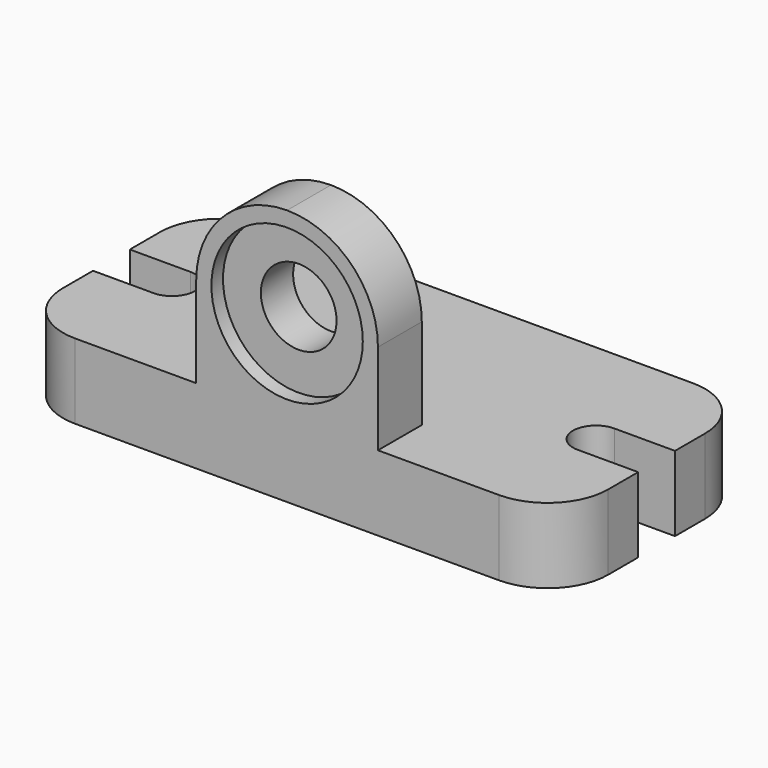
from build123d import *

# Parameters (mm, degrees)
F1_DEPTH = 15.748
F2_W     = 38.1
F2_H     = 11.4949838928
F3_DEPTH = 38.1
F4_R     = 19.04999
F6_D     = 15.875
F7_R     = 15.875
F7_R_2   = 7.9375
F8_DEPTH = 3.048


# Not quite as in the source:
# - a fillet or chamfer is up to 0.001 mm smaller than in the source, because OpenCascade refuses the exact size


with BuildPart() as f1:
    # F0 (on Top) → F1 (new body)
    with BuildSketch(Plane.XY):
        with BuildLine():
            Line((-30.7737162879, 0), (58.1262837121, 0))
            ThreePointArc((58.1262837121, 0), (67.1065398331, 3.7197438789), (70.8262837121, 12.7))
            Line((70.8262837121, 12.7), (70.8262837121, 20.574))
            Line((70.8262837121, 20.574), (58.1262837121, 20.574))
            ThreePointArc((58.1262837121, 20.574), (53.3002837121, 25.4), (58.1262837121, 30.226))
            Line((58.1262837121, 30.226), (70.8262837121, 30.226))
            Line((70.8262837121, 30.226), (70.8262837121, 38.1))
            ThreePointArc((70.8262837121, 38.1), (67.1065398331, 47.0802561211), (58.1262837121, 50.8))
            Line((58.1262837121, 50.8), (-30.7737162879, 50.8))
            ThreePointArc((-30.7737162879, 50.8), (-39.753972409, 47.0802561211), (-43.4737162879, 38.1))
            Line((-43.4737162879, 38.1), (-43.4737162879, 30.226))
            Line((-43.4737162879, 30.226), (-30.7737162879, 30.226))
            ThreePointArc((-30.7737162879, 30.226), (-25.9477162879, 25.4), (-30.7737162879, 20.574))
            Line((-30.7737162879, 20.574), (-43.4737162879, 20.574))
            Line((-43.4737162879, 20.574), (-43.4737162879, 12.7))
            ThreePointArc((-43.4737162879, 12.7), (-39.753972409, 3.7197438789), (-30.7737162879, 0))
        make_face()
    extrude(amount=F1_DEPTH)

    # F2 (on face) → F3 (join)
    with BuildSketch(Plane.XY.offset(15.748)):
        with Locations((13.6762837121, 5.7474919464)):
            Rectangle(F2_W, F2_H)
    extrude(amount=F3_DEPTH)

    # F4 (radius 19.05 in the source; OpenCascade refuses exactly that, so slightly less here)
    f4_edges = [f1.edges().sort_by_distance(p)[0] for p in [
        (-5.373716, 5.747492, 53.848),
        (32.726284, 5.747492, 53.848),
    ]]
    fillet(f4_edges, radius=F4_R)

    # F6 (through all)
    with Locations(Plane.XZ):
        with Locations((13.6762837121, 34.798)):
            Hole(F6_D / 2)

    # F7 (on face) → F8 (cut)
    with BuildSketch(Plane.XZ):
        with Locations((13.6762837121, 34.798)):
            Circle(F7_R)
        with Locations((13.6762837121, 34.798)):
            Circle(F7_R_2, mode=Mode.SUBTRACT)
    extrude(amount=-F8_DEPTH, mode=Mode.SUBTRACT)


solid = f1.part
